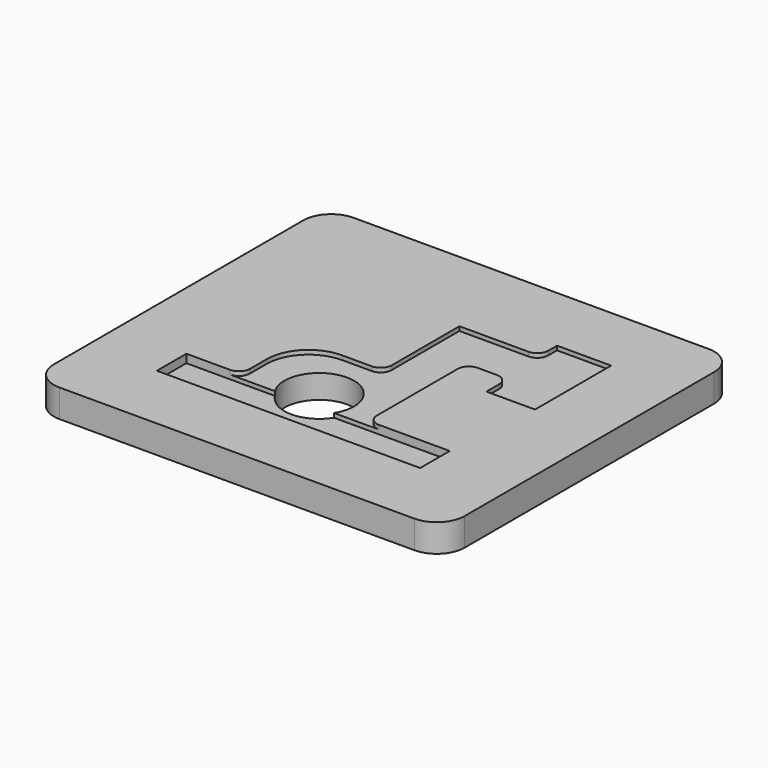
from build123d import *

# Parameters (mm, degrees)
F1_DEPTH = 4.318
F0_W     = 74.9314
F0_H     = 67.056
F2_DEPTH = 5.08
F3_DEPTH = 3.556
F4_R     = 2.032
F5_R     = 7.62
F6_R     = 5.08


# Not quite as in the source:
# - a feature names something its author has since deleted; it is built from what else it names


with BuildPart() as f1:
    # F0 (on Top) → F1 (new body)
    with BuildSketch(Plane.XY):
        with BuildLine():
            Line((2.8111794461, 24.3078), (2.8111794461, 41.656))
            Line((2.8111794461, 41.656), (-7.0454205539, 41.656))
            Line((-7.0454205539, 41.656), (-7.0454205539, 37.6428))
            Line((-7.0454205539, 37.6428), (-21.6488205539, 37.6428))
            Line((-21.6488205539, 37.6428), (-21.6488205539, 20.193))
            Line((-21.6488205539, 20.193), (-36.7380205539, 20.193))
            Line((-36.7380205539, 20.193), (-36.7380205539, 6.731))
            Line((-36.7380205539, 6.731), (-30.5658055774, 6.731))
            ThreePointArc((-30.5658055774, 6.731), (-26.9316083266, 16.200428444), (-18.8310205539, 10.0965))
            ThreePointArc((-18.8310205539, 10.0965), (-19.0770921098, 8.3459122272), (-19.7962355303, 6.731))
            Line((-19.7962355303, 6.731), (-13.6188205539, 6.731))
            Line((-13.6188205539, 6.731), (-13.6188205539, 29.2354))
            Line((-13.6188205539, 29.2354), (-6.0548205539, 29.2354))
            Line((-6.0548205539, 29.2354), (-6.0548205539, 24.3078))
            Line((-6.0548205539, 24.3078), (2.8111794461, 24.3078))
        make_face()
    extrude(amount=F1_DEPTH)

    # F0 (on Top) → F2 (join)
    with BuildSketch(Plane.XY):
        with Locations((-21.9545205539, 20.828)):
            Rectangle(F0_W, F0_H)
        Polygon((-7.0454205539, 41.656), (2.8111794461, 41.656), (2.8111794461, 24.3078), (-6.0548205539, 24.3078), (-6.0548205539, 29.2354), (-13.6188205539, 29.2354), (-13.6188205539, 6.731), (1.3111794461, 6.731), (1.3111794461, 0), (-46.7202205539, 0), (-46.7202205539, 6.731), (-36.7380205539, 6.731), (-36.7380205539, 20.193), (-21.6488205539, 20.193), (-21.6488205539, 37.6428), (-7.0454205539, 37.6428), align=None, mode=Mode.SUBTRACT)
    extrude(amount=F2_DEPTH)

    # F0 (on Top) → F3 (join)
    with BuildSketch(Plane.XY):
        with BuildLine():
            Line((1.3111794461, 6.731), (-13.6188205539, 6.731))
            Line((-13.6188205539, 6.731), (-19.7962355303, 6.731))
            ThreePointArc((-19.7962355303, 6.731), (-25.1810205539, 3.7465), (-30.5658055774, 6.731))
            Line((-30.5658055774, 6.731), (-36.7380205539, 6.731))
            Line((-36.7380205539, 6.731), (-46.7202205539, 6.731))
            Line((-46.7202205539, 6.731), (-46.7202205539, 0))
            Line((-46.7202205539, 0), (1.3111794461, 0))
            Line((1.3111794461, 0), (1.3111794461, 6.731))
        make_face()
    extrude(amount=F3_DEPTH)

    # F4
    f4_edges = [f1.edges().sort_by_distance(p)[0] for p in [
        (-7.045421, 37.6428, 4.699),
        (-13.618821, 29.2354, 4.699),
        (-21.648821, 20.193, 4.699),
        (-13.618821, 6.731, 4.699),
        (-36.738021, 6.731, 4.699),
        (-6.054821, 29.2354, 4.699),
    ]]
    fillet(f4_edges, radius=F4_R)

    # F5
    f5_edges = [f1.edges().sort_by_distance(p)[0] for p in [
        (-36.738021, 20.193, 4.699),
    ]]
    fillet(f5_edges, radius=F5_R)

    # F6
    f6_edges = [f1.edges().sort_by_distance(p)[0] for p in [
        (15.511179, -12.7, 2.54),
        (15.511179, 54.356, 2.54),
        (-59.420221, 54.356, 2.54),
        (-59.420221, -12.7, 2.54),
    ]]
    fillet(f6_edges, radius=F6_R)


solid = f1.part
